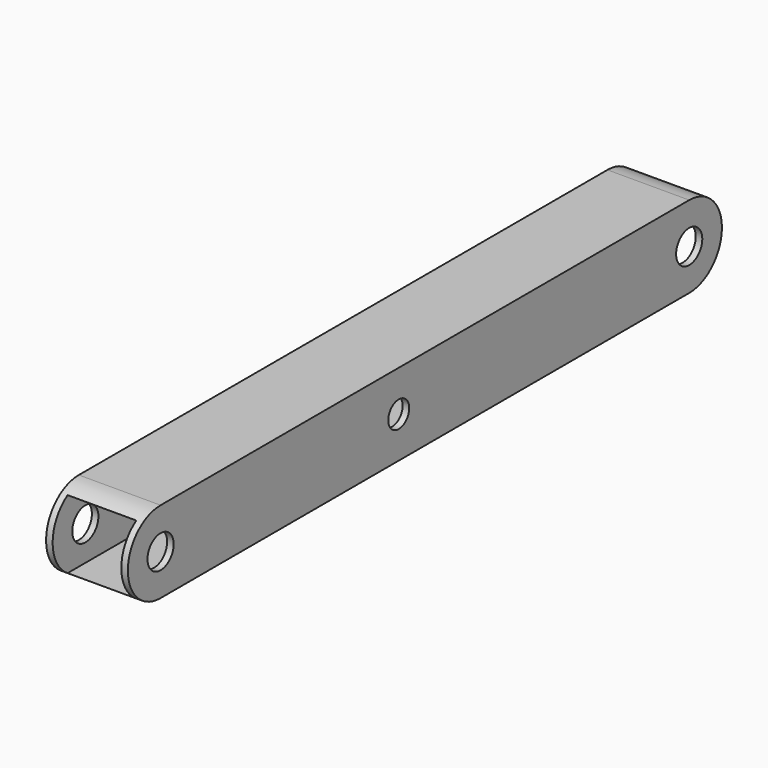
from build123d import *

# Parameters (mm, degrees)
F0_R          = 5
F0_R_2        = 4
F1_DEPTH      = 25
F2_W          = 21
F2_H          = 21
F3_DEPTH      = 113.501
F3_DEPTH_BACK = 113.501


with BuildPart() as f1:
    # F0 (on Right) → F1 (new body)
    with BuildSketch(Plane.YZ):
        with BuildLine():
            ThreePointArc((101, -12.5), (113.5, 0), (101, 12.5))
            Line((101, 12.5), (-101, 12.5))
            ThreePointArc((-101, 12.5), (-113.5, 0), (-101, -12.5))
            Line((-101, -12.5), (101, -12.5))
        make_face()
        with Locations((-101, 0)):
            Circle(F0_R, mode=Mode.SUBTRACT)
        with Locations((-10, 0)):
            Circle(F0_R_2, mode=Mode.SUBTRACT)
        with Locations((101, 0)):
            Circle(F0_R, mode=Mode.SUBTRACT)
    extrude(amount=F1_DEPTH)

    # F2 (on Front) → F3 (cut, two sides)
    with BuildSketch(Plane.XZ) as f3_sk:
        with Locations((12.5, 0)):
            Rectangle(F2_W, F2_H)
    extrude(amount=-F3_DEPTH, mode=Mode.SUBTRACT)
    extrude(f3_sk.sketch, amount=F3_DEPTH_BACK, mode=Mode.SUBTRACT)


solid = f1.part
